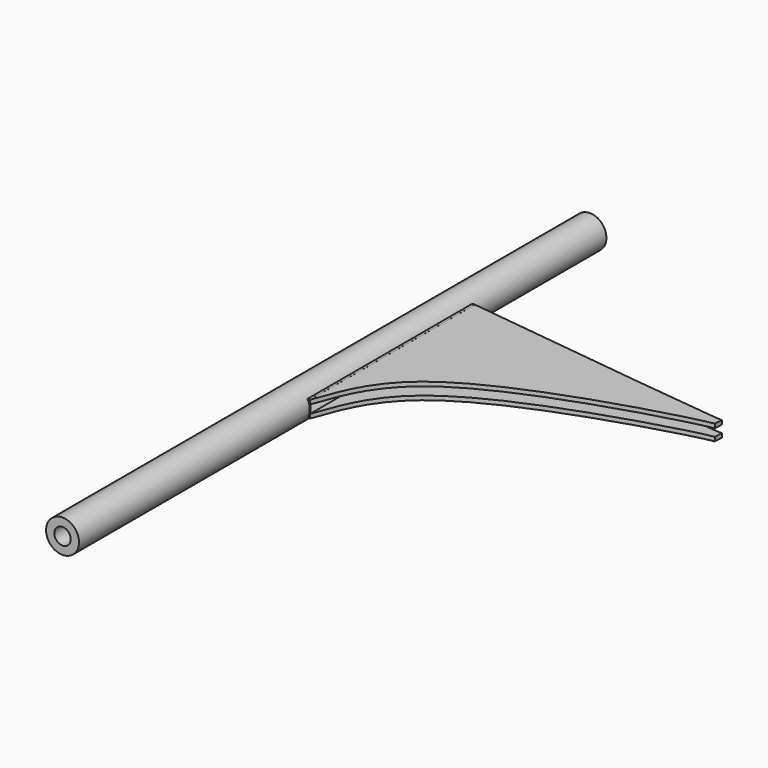
from build123d import *

# Parameters (mm, degrees)
F0_R          = 2
F0_R_2        = 1
F1_DEPTH      = 80
F5_E5_W       = 2.0043330533
F5_E5_H       = 25
F6_DEPTH      = 25
F6_DEPTH_BACK = 1
F8_W          = 25.0062048435
F8_H          = 1.0036084568
F9_DEPTH      = 0.3
F10_T         = -0.1
F12_DEPTH     = 0.5


with BuildPart() as f1:
    # F0 (on Front) → F1 (new body)
    with BuildSketch(Plane.XZ):
        Circle(F0_R)
        Circle(F0_R_2, mode=Mode.SUBTRACT)
    extrude(amount=F1_DEPTH)

    # F5_E5 (on explicit) → F6 (cut, two sides)
    with BuildSketch(Plane(origin=(0.9982800111, -45, -1.0022865608), x_dir=(-0.0038684819, 0, 0.9999925174), z_dir=(-0.9999925174, 0, -0.0038684819))) as f6_sk:
        with Locations((1.0021665267, 12.5)):
            Rectangle(F5_E5_W, F5_E5_H)
    extrude(amount=-F6_DEPTH, mode=Mode.SUBTRACT)
    extrude(f6_sk.sketch, amount=F6_DEPTH_BACK, mode=Mode.SUBTRACT)


with BuildPart() as f9:
    # F8 (on face) → F9 (new body)
    with BuildSketch(Plane(origin=(1.7307944858, 0, 0.0027212049), x_dir=(0, 1, 0), z_dir=(0.9999987641, 0, 0.0015722268))):
        with Locations((-32.4973389506, -0.5013310001)):
            Rectangle(F8_W, F8_H)
        with Locations((-32.4973389506, 0.5022774567)):
            Rectangle(F8_W, F8_H)
    extrude(amount=F9_DEPTH)

    # F10
    f10_openings = [f9.faces().sort_by_distance(p)[0] for p in [
        (2.030793, -32.497339, 0.003666),
        (1.730794, -32.497339, 0.003194),
    ]]
    offset(amount=F10_T, openings=f10_openings)


with BuildPart() as f12:
    # F11 (on face) → F12 (new body)
    with BuildSketch(Plane(origin=(0.0015771561, 0, -1.0031339887), x_dir=(0.9999987641, 0, 0.0015722268), z_dir=(0.0015722268, 0, -0.9999987641))):
        with BuildLine():
            add(Edge.make_bspline(
                [(2.030796625, 45.0004413724), (3.2768731661, 41.4614047034), (6.3001384058, 32.8748964189), (31.6399499831, 25.4198492331), (34.290238067, 24.9098338007), (34.9821001291, 24.7766934335)],
                knots=[0, 0, 0, 0, 0.3412879074, 0.8280421251, 1, 1, 1, 1], degree=3))
            Line((2.030796625, 45.0004413724), (2.030796625, 19.9942365289))
            add(Edge.make_bspline(
                [(2.030796625, 19.9942365289), (18.4971969643, 21.9813155341), (34.9635973036, 23.9683945393), (35.0341200829, 23.7715635449)],
                knots=[0, 0, 0, 0, 0.9586021312, 0.9586021312, 0.9586021312, 0.9586021312], degree=3))
            Line((35.0341200829, 23.7715635449), (34.9821001291, 24.7766934335))
        make_face()
    extrude(amount=-F12_DEPTH)


with BuildPart() as f14_1:
    # F14: instance of F12
    add(f12.part.mirror(Plane.XY.offset(0.0031944326)))


solid = Compound([f1.part, f9.part, f12.part, f14_1.part])
